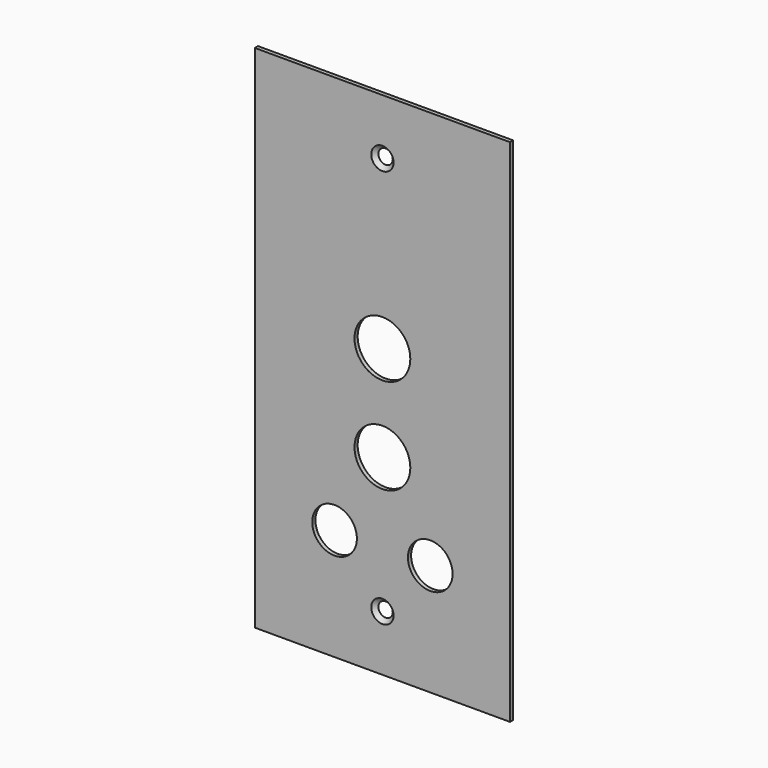
from build123d import *

# Parameters (mm, degrees)
F0_W     = 160
F0_H     = 320
F0_R     = 14
F0_R_2   = 3
F0_R_3   = 17.5
F1_DEPTH = 2.5


# Not quite as in the source:
# - a fillet or chamfer that OpenCascade refuses, or shapes differently, is made with other operations: its cross-section is extruded or revolved along the edge and cut away or added


with BuildPart() as f1:
    # F0 (on Front) → F1 (new body)
    with BuildSketch(Plane.XZ):
        with Locations((-1.8876045942, 29.6809725389)):
            Rectangle(F0_W, F0_H)
        with Locations((-31.8876045942, -60.3190274611)):
            Circle(F0_R, mode=Mode.SUBTRACT)
        with Locations((-1.8876045942, -95.3190274611)):
            Circle(F0_R_2, mode=Mode.SUBTRACT)
        with Locations((28.1123954058, -60.3190274611)):
            Circle(F0_R, mode=Mode.SUBTRACT)
        with Locations((-1.8876045942, -10.3190274611)):
            Circle(F0_R_3, mode=Mode.SUBTRACT)
        with Locations((-1.8876045942, 49.6809725389)):
            Circle(F0_R_3, mode=Mode.SUBTRACT)
        with Locations((-1.8876045942, 154.6809725389)):
            Circle(F0_R_2, mode=Mode.SUBTRACT)
    extrude(amount=F1_DEPTH)

    # F2: chamfer of 4 on 2 edges, made by hand

    # F2_s1 → F2_t2 (revolve, cut)
    with BuildSketch(Plane.XY.offset(154.6809725389)):
        Polygon((1.1123954058, 1.5), (5.1123954058, -2.5), (1.1123954058, -2.5), align=None)
    revolve(axis=Axis((-1.8876045942, -2.5, 154.6809725389), (0, -1, 0)), mode=Mode.SUBTRACT)

    # F2_s3 → F2_t4 (revolve, cut)
    with BuildSketch(Plane.XY.offset(-95.3190274611)):
        Polygon((1.1123954058, 1.5), (5.1123954058, -2.5), (1.1123954058, -2.5), align=None)
    revolve(axis=Axis((-1.8876045942, -2.5, -95.3190274611), (0, -1, 0)), mode=Mode.SUBTRACT)


solid = f1.part
